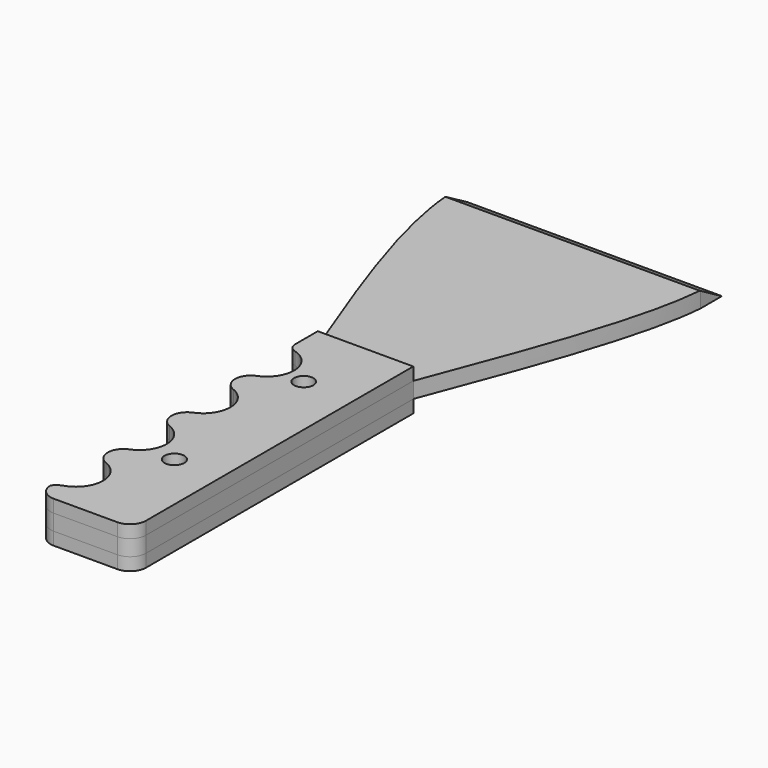
from build123d import *

# Parameters (mm, degrees)
F0_W        = 30
F0_H        = 90
F0_H_2      = 110
F1_DEPTH    = 5
F3_R        = 5
F4_DEPTH    = 25
F5_T1_DEPTH = 25.1996810199
F5_T3_DEPTH = 18.0610213145
F6_R        = 3
F7_SIZE2    = 8.660244
F7_SIZE     = 4.99999
F9_DEPTH    = 4
F11_DEPTH   = 4
F12_R       = 3.0392347024
F12_R_2     = 3.1
F13_DEPTH   = 25


# Not quite as in the source:
# - a fillet or chamfer that OpenCascade refuses, or shapes differently, is made with other operations: its cross-section is extruded or revolved along the edge and cut away or added
# - a fillet or chamfer is up to 0.001 mm smaller than in the source, because OpenCascade refuses the exact size


with BuildPart() as f1:
    # F0 (on Top) → F1 (new body)
    with BuildSketch(Plane.XY):
        with BuildLine():
            add(Edge.make_bspline(
                [(-11.2144336104, 57.1776708961), (-22.912006026, 87.7576573075), (-34.6095784415, 118.3376437189), (-36.2144336104, 138.6793877413)],
                knots=[0, 0, 0, 0, 0.5742115835, 0.5742115835, 0.5742115835, 0.5742115835], degree=3))
            Line((-11.2144336104, 57.1776708961), (-11.2144336104, 147.1776708961))
            Line((-11.2144336104, 147.1776708961), (-36.2144336104, 147.1776708961))
            Line((-36.2144336104, 147.1776708961), (-36.2144336104, 138.6793877413))
        make_face()
        with Locations((3.7855663896, 102.1776708961)):
            Rectangle(F0_W, F0_H)
        with BuildLine():
            Line((18.7855663896, 147.1776708961), (18.7855663896, 57.1776708961))
            add(Edge.make_bspline(
                [(18.7855663896, 57.1776708961), (30.4925554698, 87.8723420853), (42.1995445501, 118.5670132745), (43.7855663896, 138.8334699858)],
                knots=[0, 0, 0, 0, 0.5773994274, 0.5773994274, 0.5773994274, 0.5773994274], degree=3))
            Line((43.7855663896, 138.8334699858), (43.7855663896, 147.1776708961))
            Line((43.7855663896, 147.1776708961), (18.7855663896, 147.1776708961))
        make_face()
        with Locations((3.7855663896, 2.1776708961)):
            Rectangle(F0_W, F0_H_2)
    extrude(amount=F1_DEPTH)

    # F3
    f3_edges = [f1.edges().sort_by_distance(p)[0] for p in [
        (-11.214434, -52.822329, 2.5),
        (18.785566, -52.822329, 2.5),
    ]]
    fillet(f3_edges, radius=F3_R)

    # F2 (on face) → F4 (cut)
    with BuildSketch(Plane.XY.offset(5)):
        with BuildLine():
            ThreePointArc((-11.2144336104, 28.6776708961), (-5.2040259704, 31.167263256), (-2.7144336104, 37.1776708961))
            ThreePointArc((-2.7144336104, 37.1776708961), (-5.2040259704, 43.1880785361), (-11.2144336104, 45.6776708961))
            Line((-11.2144336104, 45.6776708961), (-11.2144336104, 28.6776708961))
        make_face()
        with BuildLine():
            ThreePointArc((-2.7144336104, 12.1776708961), (-5.2040259704, 18.1880785361), (-11.2144336104, 20.6776708961))
            Line((-11.2144336104, 20.6776708961), (-11.2144336104, 3.6776708961))
            ThreePointArc((-11.2144336104, 3.6776708961), (-5.2040259704, 6.167263256), (-2.7144336104, 12.1776708961))
        make_face()
        with BuildLine():
            ThreePointArc((-2.7144336104, -12.8223291039), (-5.2040259704, -6.8119214639), (-11.2144336104, -4.3223291039))
            Line((-11.2144336104, -4.3223291039), (-11.2144336104, -21.3223291039))
            ThreePointArc((-11.2144336104, -21.3223291039), (-5.2040259704, -18.832736744), (-2.7144336104, -12.8223291039))
        make_face()
        with BuildLine():
            ThreePointArc((-2.7144336104, -37.8223291039), (-5.2040259704, -31.8119214639), (-11.2144336104, -29.3223291039))
            Line((-11.2144336104, -29.3223291039), (-11.2144336104, -46.3223291039))
            ThreePointArc((-11.2144336104, -46.3223291039), (-5.2040259704, -43.832736744), (-2.7144336104, -37.8223291039))
        make_face()
    extrude(amount=-F4_DEPTH, mode=Mode.SUBTRACT)

    # F5: fillet of radius 5 on 7 edges, made by hand

    # F5_s2 → F5_t1 (cut)
    with BuildSketch(Plane.XY.offset(-10.09984051)):
        with BuildLine():
            ThreePointArc((-11.2144336104, -0.2823929), (-10.3532292843, -3.0878109384), (-8.0662854623, -4.9268137163))
            ThreePointArc((-8.0662854623, -4.9268137163), (-9.6116049851, -4.4748180738), (-11.2144336104, -4.3223291039))
            Line((-11.2144336104, -4.3223291039), (-11.2144336104, -0.2823929))
        make_face()
        with BuildLine():
            ThreePointArc((-8.0662854623, 4.2821555084), (-10.3532292843, 2.4431527305), (-11.2144336104, -0.3622653079))
            Line((-11.2144336104, -0.3622653079), (-11.2144336104, 3.6776708961))
            ThreePointArc((-11.2144336104, 3.6776708961), (-9.6116049851, 3.8301598659), (-8.0662854623, 4.2821555084))
        make_face()
        with BuildLine():
            ThreePointArc((-8.0662854623, -20.7178444916), (-10.3532292843, -22.5568472695), (-11.2144336104, -25.3622653079))
            Line((-11.2144336104, -25.3622653079), (-11.2144336104, -21.3223291039))
            ThreePointArc((-11.2144336104, -21.3223291039), (-9.6116049851, -21.1698401341), (-8.0662854623, -20.7178444916))
        make_face()
        with BuildLine():
            ThreePointArc((-11.2144336104, -25.2823929), (-10.3532292843, -28.0878109384), (-8.0662854623, -29.9268137163))
            ThreePointArc((-8.0662854623, -29.9268137163), (-9.6116049851, -29.4748180738), (-11.2144336104, -29.3223291039))
            Line((-11.2144336104, -29.3223291039), (-11.2144336104, -25.2823929))
        make_face()
        with BuildLine():
            ThreePointArc((-11.2144336104, 24.7176071), (-10.3532292843, 21.9121890616), (-8.0662854623, 20.0731862837))
            ThreePointArc((-8.0662854623, 20.0731862837), (-9.6116049851, 20.5251819262), (-11.2144336104, 20.6776708961))
            Line((-11.2144336104, 20.6776708961), (-11.2144336104, 24.7176071))
        make_face()
        with BuildLine():
            ThreePointArc((-8.0662854623, 29.2821555084), (-10.3532292843, 27.4431527305), (-11.2144336104, 24.6377346921))
            Line((-11.2144336104, 24.6377346921), (-11.2144336104, 28.6776708961))
            ThreePointArc((-11.2144336104, 28.6776708961), (-9.6116049851, 28.8301598659), (-8.0662854623, 29.2821555084))
        make_face()
    extrude(amount=F5_T1_DEPTH, mode=Mode.SUBTRACT)

    # F5_s4 → F5_t3 (cut)
    with BuildSketch(Plane.XY.offset(-6.5305106572)):
        with BuildLine():
            ThreePointArc((-8.6332520843, -45.9209402151), (-10.0803650529, -46.6591519697), (-11.2144336104, -47.8223291039))
            Line((-11.2144336104, -47.8223291039), (-11.2144336104, -46.3223291039))
            ThreePointArc((-11.2144336104, -46.3223291039), (-9.908331479, -46.2213824567), (-8.6332520843, -45.9209402151))
        make_face()
    extrude(amount=F5_T3_DEPTH, mode=Mode.SUBTRACT)

    # F6
    f6_edges = [f1.edges().sort_by_distance(p)[0] for p in [
        (-11.214434, 45.677671, 2.5),
    ]]
    fillet(f6_edges, radius=F6_R)

    # F7 (size 5 and 8.6602540378 in the source; OpenCascade refuses exactly that, so slightly less here)
    f7_edges = [f1.edges().sort_by_distance(p)[0] for p in [
        (3.785566, 147.177671, 5),
    ]]
    f7_side = f1.faces().sort_by_distance((3.785566, 147.177671, 2.5))[0]
    chamfer(f7_edges, length=F7_SIZE, length2=F7_SIZE2, reference=f7_side)


with BuildPart() as f9:
    # F8 (on face) → F9 (new body)
    with BuildSketch(Plane.XY.offset(5)):
        with BuildLine():
            Line((18.7855663896, 57.1776708961), (-11.2144336104, 57.1776708961))
            Line((-11.2144336104, 57.1776708961), (-11.2144336104, 48.2794725516))
            ThreePointArc((-11.2144336104, 48.2794725516), (-10.5964313106, 46.455716275), (-8.9970423061, 45.3833503806))
            ThreePointArc((-8.9970423061, 45.3833503806), (-2.7285999753, 37.6682088837), (-8.0662854623, 29.2821555084))
            ThreePointArc((-8.0662854623, 29.2821555084), (-10.3419924147, 27.4596592689), (-11.2142741178, 24.677670896))
            ThreePointArc((-11.2142741178, 24.677670896), (-10.3419924147, 21.8956825232), (-8.0662854623, 20.0731862837))
            ThreePointArc((-8.0662854623, 20.0731862837), (-2.7144336104, 12.1776708961), (-8.0662854623, 4.2821555084))
            ThreePointArc((-8.0662854623, 4.2821555084), (-10.3419924147, 2.4596592689), (-11.2142741178, -0.322329104))
            ThreePointArc((-11.2142741178, -0.322329104), (-10.3419924147, -3.1043174768), (-8.0662854623, -4.9268137163))
            ThreePointArc((-8.0662854623, -4.9268137163), (-2.7144336104, -12.8223291039), (-8.0662854623, -20.7178444916))
            ThreePointArc((-8.0662854623, -20.7178444916), (-10.3419924147, -22.5403407311), (-11.2142741178, -25.322329104))
            ThreePointArc((-11.2142741178, -25.322329104), (-10.3419924147, -28.1043174768), (-8.0662854623, -29.9268137163))
            ThreePointArc((-8.0662854623, -29.9268137163), (-2.7197690942, -38.123451597), (-8.6332520843, -45.9209402151))
            ThreePointArc((-8.6332520843, -45.9209402151), (-10.0803650529, -46.6591519697), (-11.2144336104, -47.8223291039))
            ThreePointArc((-11.2144336104, -47.8223291039), (-9.7499675164, -51.3578630099), (-6.2144336104, -52.8223291039))
            Line((-6.2144336104, -52.8223291039), (13.7855663896, -52.8223291039))
            ThreePointArc((13.7855663896, -52.8223291039), (17.3211002955, -51.3578630099), (18.7855663896, -47.8223291039))
            Line((18.7855663896, -47.8223291039), (18.7855663896, 57.1776708961))
        make_face()
    extrude(amount=F9_DEPTH)


with BuildPart() as f11:
    # F10 (on face) → F11 (new body)
    with BuildSketch(Plane(origin=(0, 0, 0), x_dir=(1, 0, 0), z_dir=(0, 0, -1))):
        with BuildLine():
            Line((-11.2144336104, -57.1776708961), (18.7855663896, -57.1776708961))
            Line((18.7855663896, -57.1776708961), (18.7855663896, 47.8223291039))
            ThreePointArc((18.7855663896, 47.8223291039), (17.3211002955, 51.3578630099), (13.7855663896, 52.8223291039))
            Line((13.7855663896, 52.8223291039), (-6.2144336104, 52.8223291039))
            ThreePointArc((-6.2144336104, 52.8223291039), (-9.7499675164, 51.3578630099), (-11.2144336104, 47.8223291039))
            ThreePointArc((-11.2144336104, 47.8223291039), (-10.0803650529, 46.6591519697), (-8.6332520843, 45.9209402151))
            ThreePointArc((-8.6332520843, 45.9209402151), (-2.7197690942, 38.123451597), (-8.0662854623, 29.9268137163))
            ThreePointArc((-8.0662854623, 29.9268137163), (-10.3419924147, 28.1043174768), (-11.2142741178, 25.322329104))
            ThreePointArc((-11.2142741178, 25.322329104), (-10.3419924147, 22.5403407311), (-8.0662854623, 20.7178444916))
            ThreePointArc((-8.0662854623, 20.7178444916), (-2.7144336104, 12.8223291039), (-8.0662854623, 4.9268137163))
            ThreePointArc((-8.0662854623, 4.9268137163), (-10.3419924147, 3.1043174768), (-11.2142741178, 0.322329104))
            ThreePointArc((-11.2142741178, 0.322329104), (-10.3419924147, -2.4596592689), (-8.0662854623, -4.2821555084))
            ThreePointArc((-8.0662854623, -4.2821555084), (-2.7144336104, -12.1776708961), (-8.0662854623, -20.0731862837))
            ThreePointArc((-8.0662854623, -20.0731862837), (-10.3419924147, -21.8956825232), (-11.2142741178, -24.677670896))
            ThreePointArc((-11.2142741178, -24.677670896), (-10.3419924147, -27.4596592689), (-8.0662854623, -29.2821555084))
            ThreePointArc((-8.0662854623, -29.2821555084), (-2.7285999753, -37.6682088837), (-8.9970423061, -45.3833503806))
            ThreePointArc((-8.9970423061, -45.3833503806), (-10.5964313106, -46.455716275), (-11.2144336104, -48.2794725516))
            Line((-11.2144336104, -48.2794725516), (-11.2144336104, -57.1776708961))
        make_face()
    extrude(amount=F11_DEPTH)


with BuildPart() as f13_tool:
    # F12 (on face) → F13 (new body)
    with BuildSketch(Plane.XY.offset(9)):
        with Locations((2.841765537, 34.0852281909)):
            Circle(F12_R)
        with Locations((3.8561289876, -17.9932220587)):
            Circle(F12_R_2)
    extrude(amount=-F13_DEPTH)


with BuildPart() as f1_1:
    add(f1.part)

    # F13: cut by f13_tool
    add(f13_tool.part, mode=Mode.SUBTRACT)


with BuildPart() as f9_1:
    add(f9.part)

    # F13: cut by f13_tool
    add(f13_tool.part, mode=Mode.SUBTRACT)


with BuildPart() as f11_1:
    add(f11.part)

    # F13: cut by f13_tool
    add(f13_tool.part, mode=Mode.SUBTRACT)


solid = Compound([f1_1.part, f9_1.part, f11_1.part])
